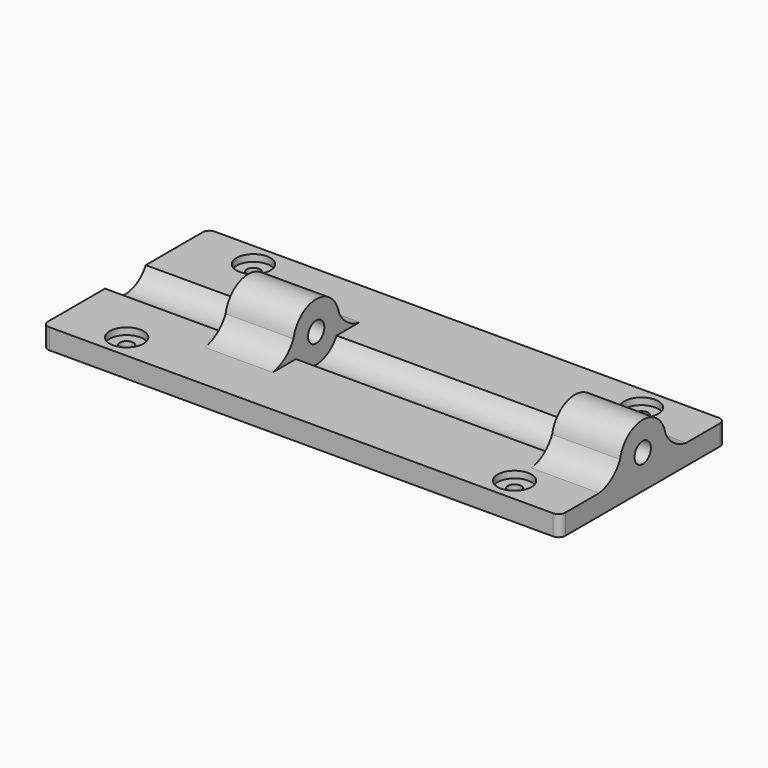
from build123d import *

# Parameters (mm, degrees)
F0_W          = 76.2
F0_H          = 30.48
F0_R          = 2.5
F2_DEPTH      = 3
F0_R_2        = 1
F3_DEPTH      = 2
F4_START      = 28.1
F1_R          = 1.5
F4_DEPTH      = 10
F5_START      = -10
F5_DEPTH      = 10
F6_DEPTH      = 10
F6_DEPTH_BACK = 28.1
F7_R          = 1
F8_START      = -20
F8_DEPTH      = 30


with BuildPart() as f2:
    # F0 (on Top) → F2 (new body)
    with BuildSketch(Plane.XY):
        with Locations((0, 1.624652555)):
            Rectangle(F0_W, F0_H)
        with Locations((-28.57, -10.055347445)):
            Circle(F0_R, mode=Mode.SUBTRACT)
        with Locations((28.57, -10.055347445)):
            Circle(F0_R, mode=Mode.SUBTRACT)
        with Locations((-28.57, 13.304652555)):
            Circle(F0_R, mode=Mode.SUBTRACT)
        with Locations((28.57, 13.304652555)):
            Circle(F0_R, mode=Mode.SUBTRACT)
    extrude(amount=F2_DEPTH)

    # F0 (on Top) → F3 (join)
    with BuildSketch(Plane.XY):
        with Locations((28.57, 13.304652555)):
            Circle(F0_R)
        with Locations((28.57, 13.304652555)):
            Circle(F0_R_2, mode=Mode.SUBTRACT)
        with Locations((28.57, -10.055347445)):
            Circle(F0_R)
        with Locations((28.57, -10.055347445)):
            Circle(F0_R_2, mode=Mode.SUBTRACT)
        with Locations((-28.57, -10.055347445)):
            Circle(F0_R)
        with Locations((-28.57, -10.055347445)):
            Circle(F0_R_2, mode=Mode.SUBTRACT)
        with Locations((-28.57, 13.304652555)):
            Circle(F0_R)
        with Locations((-28.57, 13.304652555)):
            Circle(F0_R_2, mode=Mode.SUBTRACT)
    extrude(amount=F3_DEPTH)

    # F1 (on Right) → F4 (join)
    with BuildSketch(Plane.YZ.offset(F4_START)):
        with BuildLine():
            ThreePointArc((-2.5401260508, 5.7960675804), (-4.1005061168, 3.9161569732), (-6.365347445, 3))
            Line((-6.365347445, 3), (-2.115347445, 3))
            ThreePointArc((-2.115347445, 3), (-2.5671360482, 4.3616642469), (-2.5401260508, 5.7960675804))
        make_face()
        with BuildLine():
            Line((5.384652555, 3), (9.634652555, 3))
            ThreePointArc((9.634652555, 3), (7.3698112268, 3.9161569732), (5.8094311608, 5.7960675804))
            ThreePointArc((5.8094311608, 5.7960675804), (5.8658054165, 5.3998067817), (5.884652555, 5))
            ThreePointArc((5.884652555, 5), (5.7577581806, 3.9692235936), (5.384652555, 3))
        make_face()
        with BuildLine():
            ThreePointArc((-2.5401260508, 5.7960675804), (-2.5671360482, 4.3616642469), (-2.115347445, 3))
            Line((-2.115347445, 3), (5.384652555, 3))
            ThreePointArc((5.384652555, 3), (5.7577581806, 3.9692235936), (5.884652555, 5))
            ThreePointArc((5.884652555, 5), (5.8658054165, 5.3998067817), (5.8094311608, 5.7960675804))
            ThreePointArc((5.8094311608, 5.7960675804), (1.634652555, 9.25), (-2.5401260508, 5.7960675804))
        make_face()
        with Locations((1.634652555, 5)):
            Circle(F1_R, mode=Mode.SUBTRACT)
    extrude(amount=F4_DEPTH)

    # F1 (on Right) → F5 (join)
    with BuildSketch(Plane.YZ.offset(F5_START)):
        with BuildLine():
            ThreePointArc((-2.5401260508, 5.7960675804), (-4.1005061168, 3.9161569732), (-6.365347445, 3))
            Line((-6.365347445, 3), (-2.115347445, 3))
            ThreePointArc((-2.115347445, 3), (-2.5671360482, 4.3616642469), (-2.5401260508, 5.7960675804))
        make_face()
        with BuildLine():
            Line((5.384652555, 3), (9.634652555, 3))
            ThreePointArc((9.634652555, 3), (7.3698112268, 3.9161569732), (5.8094311608, 5.7960675804))
            ThreePointArc((5.8094311608, 5.7960675804), (5.8658054165, 5.3998067817), (5.884652555, 5))
            ThreePointArc((5.884652555, 5), (5.7577581806, 3.9692235936), (5.384652555, 3))
        make_face()
        with BuildLine():
            ThreePointArc((-2.5401260508, 5.7960675804), (-2.5671360482, 4.3616642469), (-2.115347445, 3))
            Line((-2.115347445, 3), (5.384652555, 3))
            ThreePointArc((5.384652555, 3), (5.7577581806, 3.9692235936), (5.884652555, 5))
            ThreePointArc((5.884652555, 5), (5.8658054165, 5.3998067817), (5.8094311608, 5.7960675804))
            ThreePointArc((5.8094311608, 5.7960675804), (1.634652555, 9.25), (-2.5401260508, 5.7960675804))
        make_face()
        with Locations((1.634652555, 5)):
            Circle(F1_R, mode=Mode.SUBTRACT)
    extrude(amount=-F5_DEPTH)

    # F1 (on Right) → F6 (cut, two sides)
    with BuildSketch(Plane.YZ) as f6_sk:
        with BuildLine():
            Line((5.384652555, 3), (-2.115347445, 3))
            ThreePointArc((-2.115347445, 3), (1.634652555, 0.75), (5.384652555, 3))
        make_face()
    extrude(amount=-F6_DEPTH, mode=Mode.SUBTRACT)
    extrude(f6_sk.sketch, amount=F6_DEPTH_BACK, mode=Mode.SUBTRACT)

    # F7
    f7_edges = [f2.edges().sort_by_distance(p)[0] for p in [
        (38.1, -13.615347, 1.5),
        (38.1, 16.864653, 1.5),
        (-38.1, 16.864653, 1.5),
        (-38.1, -13.615347, 1.5),
    ]]
    fillet(f7_edges, radius=F7_R)

    # F1 (on Right) → F8 (cut)
    with BuildSketch(Plane.YZ.offset(F8_START)):
        with BuildLine():
            ThreePointArc((-2.5401260508, 5.7960675804), (-2.5671360482, 4.3616642469), (-2.115347445, 3))
            Line((-2.115347445, 3), (5.384652555, 3))
            ThreePointArc((5.384652555, 3), (5.7577581806, 3.9692235936), (5.884652555, 5))
            ThreePointArc((5.884652555, 5), (5.8658054165, 5.3998067817), (5.8094311608, 5.7960675804))
            ThreePointArc((5.8094311608, 5.7960675804), (1.634652555, 9.25), (-2.5401260508, 5.7960675804))
        make_face()
        with Locations((1.634652555, 5)):
            Circle(F1_R, mode=Mode.SUBTRACT)
        with BuildLine():
            Line((5.384652555, 3), (-2.115347445, 3))
            ThreePointArc((-2.115347445, 3), (1.634652555, 0.75), (5.384652555, 3))
        make_face()
    extrude(amount=-F8_DEPTH, mode=Mode.SUBTRACT)


solid = f2.part
